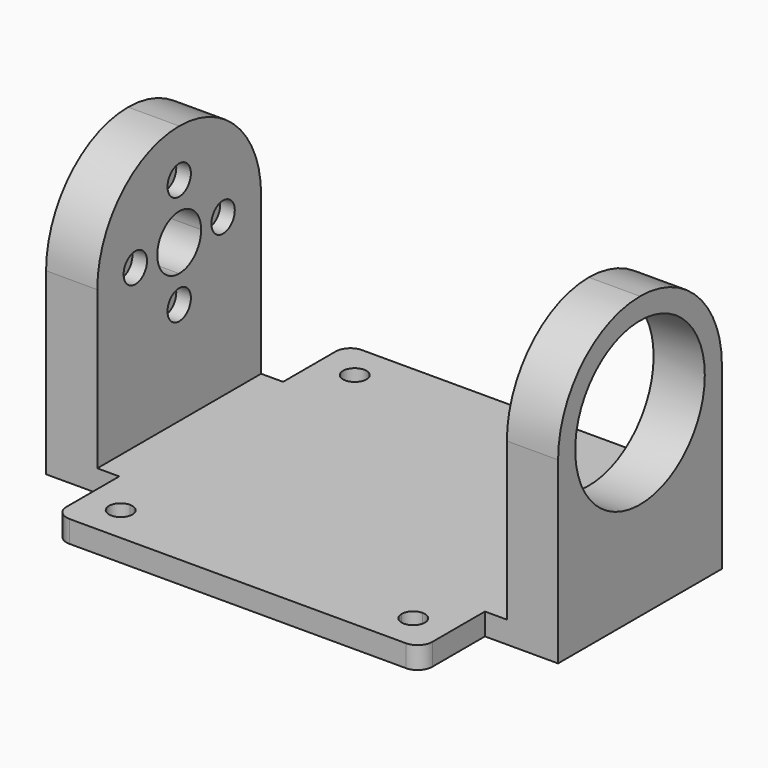
from build123d import *

# Parameters (mm, degrees)
F0_W      = 10
F0_H      = 14
F1_DEPTH  = 3
F2_W      = 7
F2_H      = 28
F3_DEPTH  = 35.5
F5_DEPTH  = 70.001
F6_R      = 11.075
F7_DEPTH  = 7
F9_DEPTH  = 25
F10_R     = 2
F11_DEPTH = 2


with BuildPart() as f1:
    # F0 (on Top) → F1 (new body)
    with BuildSketch(Plane.XY):
        with BuildLine():
            ThreePointArc((25, 23), (24.4142135624, 24.4142135624), (23, 25))
            Line((23, 25), (-23, 25))
            ThreePointArc((-23, 25), (-24.4142135624, 24.4142135624), (-25, 23))
            Line((-25, 23), (-25, 14))
            Line((-25, 14), (-25, 0))
            Line((-25, 0), (-25, -14))
            Line((-25, -14), (-25, -23))
            ThreePointArc((-25, -23), (-24.4142135624, -24.4142135624), (-23, -25))
            Line((-23, -25), (23, -25))
            ThreePointArc((23, -25), (24.4142135624, -24.4142135624), (25, -23))
            Line((25, -23), (25, -14))
            Line((25, -14), (25, 0))
            Line((25, 0), (25, 14))
            Line((25, 14), (25, 23))
        make_face()
        with BuildLine():
            ThreePointArc((-20, 18.4), (-21.1313708499, 21.1313708499), (-18.4, 20))
            Line((-18.4, 20), (18.4, 20))
            ThreePointArc((18.4, 20), (20, 21.6), (21.6, 20))
            ThreePointArc((21.6, 20), (21.1313708499, 18.8686291501), (20, 18.4))
            Line((20, 18.4), (20, -18.4))
            ThreePointArc((20, -18.4), (21.1313708499, -18.8686291501), (21.6, -20))
            ThreePointArc((21.6, -20), (20, -21.6), (18.4, -20))
            Line((18.4, -20), (-18.4, -20))
            ThreePointArc((-18.4, -20), (-21.1313708499, -21.1313708499), (-20, -18.4))
            Line((-20, -18.4), (-20, 18.4))
        make_face(mode=Mode.SUBTRACT)
        with Locations((30, 7)):
            Rectangle(F0_W, F0_H)
        with Locations((-30, 7)):
            Rectangle(F0_W, F0_H)
        with Locations((30, -7)):
            Rectangle(F0_W, F0_H)
        with Locations((-30, -7)):
            Rectangle(F0_W, F0_H)
        with BuildLine():
            Line((18.4, 20), (-18.4, 20))
            ThreePointArc((-18.4, 20), (-18.8686291501, 18.8686291501), (-20, 18.4))
            Line((-20, 18.4), (-20, -18.4))
            ThreePointArc((-20, -18.4), (-18.8686291501, -18.8686291501), (-18.4, -20))
            Line((-18.4, -20), (18.4, -20))
            ThreePointArc((18.4, -20), (18.8686291501, -18.8686291501), (20, -18.4))
            Line((20, -18.4), (20, 18.4))
            ThreePointArc((20, 18.4), (18.8686291501, 18.8686291501), (18.4, 20))
        make_face()
    extrude(amount=F1_DEPTH)

    # F2 (on face) → F3 (join)
    with BuildSketch(Plane.XY.offset(3)):
        with Locations((-31.5, 0)):
            Rectangle(F2_W, F2_H)
        with Locations((31.5, 0)):
            Rectangle(F2_W, F2_H)
    extrude(amount=F3_DEPTH)

    # F4 (on face) → F5 (cut, through all)
    with BuildSketch(Plane(origin=(-35, 0, 0), x_dir=(0, -1, 0), z_dir=(-1, 0, 0))):
        with BuildLine():
            Line((14, 38.5), (0, 38.5))
            ThreePointArc((0, 38.5), (9.8994949366, 34.3994949366), (14, 24.5))
            Line((14, 24.5), (14, 38.5))
        make_face()
        with BuildLine():
            ThreePointArc((-14, 24.5), (-9.8994949366, 34.3994949366), (0, 38.5))
            Line((0, 38.5), (-14, 38.5))
            Line((-14, 38.5), (-14, 24.5))
        make_face()
    extrude(amount=-F5_DEPTH, mode=Mode.SUBTRACT)

    # F6 (on face) → F7 (cut, through all)
    with BuildSketch(Plane.YZ.offset(35)):
        with Locations((0, 24.5)):
            Circle(F6_R)
    extrude(amount=-F7_DEPTH, mode=Mode.SUBTRACT)

    # F8 (on face) → F9 (cut)
    with BuildSketch(Plane(origin=(-35, 0, 0), x_dir=(0, -1, 0), z_dir=(-1, 0, 0))):
        with BuildLine():
            ThreePointArc((1, 32), (0.7071067812, 32.7071067812), (0, 33))
            Line((0, 33), (0, 32))
            ThreePointArc((0, 32), (0.5, 31.9833147735), (0.9977753031, 31.9333333333))
            ThreePointArc((0.9977753031, 31.9333333333), (0.999443671, 31.966648112), (1, 32))
        make_face()
        with BuildLine():
            Line((0, 32), (0, 33))
            ThreePointArc((0, 33), (-0.7302967433, 32.6831300511), (-0.9977753031, 31.9333333333))
            ThreePointArc((-0.9977753031, 31.9333333333), (-0.5, 31.9833147735), (0, 32))
        make_face()
        with BuildLine():
            Line((0, 31), (0, 32))
            ThreePointArc((0, 32), (-0.5, 31.9833147735), (-0.9977753031, 31.9333333333))
            ThreePointArc((-0.9977753031, 31.9333333333), (-0.6831300511, 31.2697032567), (0, 31))
        make_face()
        with BuildLine():
            ThreePointArc((0.9977753031, 31.9333333333), (0.5, 31.9833147735), (0, 32))
            Line((0, 32), (0, 31))
            ThreePointArc((0, 31), (0.6831300511, 31.2697032567), (0.9977753031, 31.9333333333))
        make_face()
        with BuildLine():
            ThreePointArc((-6.5, 24.5), (-6.7697032567, 25.1831300511), (-7.4333333333, 25.4977753031))
            ThreePointArc((-7.4333333333, 25.4977753031), (-7.4833147735, 25), (-7.5, 24.5))
            Line((-7.5, 24.5), (-6.5, 24.5))
        make_face()
        with BuildLine():
            ThreePointArc((-7.5, 24.5), (-7.4833147735, 25), (-7.4333333333, 25.4977753031))
            ThreePointArc((-7.4333333333, 25.4977753031), (-8.5, 24.5), (-7.4333333333, 23.5022246969))
            ThreePointArc((-7.4333333333, 23.5022246969), (-7.4833147735, 24), (-7.5, 24.5))
        make_face()
        with BuildLine():
            ThreePointArc((8.5, 24.5), (8.1831300511, 25.2302967433), (7.4333333333, 25.4977753031))
            ThreePointArc((7.4333333333, 25.4977753031), (7.4833147735, 25), (7.5, 24.5))
            ThreePointArc((7.5, 24.5), (7.4833147735, 24), (7.4333333333, 23.5022246969))
            ThreePointArc((7.4333333333, 23.5022246969), (8.1831300511, 23.7697032567), (8.5, 24.5))
        make_face()
        with BuildLine():
            ThreePointArc((7.5, 24.5), (7.4833147735, 25), (7.4333333333, 25.4977753031))
            ThreePointArc((7.4333333333, 25.4977753031), (6.7697032567, 25.1831300511), (6.5, 24.5))
            Line((6.5, 24.5), (7.5, 24.5))
        make_face()
        with BuildLine():
            ThreePointArc((3.75, 24.5), (2.6516504294, 27.1516504294), (0, 28.25))
            Line((0, 28.25), (0, 24.5))
            Line((0, 24.5), (3.75, 24.5))
        make_face()
        with BuildLine():
            Line((0, 24.5), (0, 28.25))
            ThreePointArc((0, 28.25), (-2.6516504294, 27.1516504294), (-3.75, 24.5))
            Line((-3.75, 24.5), (0, 24.5))
        make_face()
        with BuildLine():
            Line((-6.5, 24.5), (-7.5, 24.5))
            ThreePointArc((-7.5, 24.5), (-7.4833147735, 24), (-7.4333333333, 23.5022246969))
            ThreePointArc((-7.4333333333, 23.5022246969), (-6.7697032567, 23.8168699489), (-6.5, 24.5))
        make_face()
        with BuildLine():
            ThreePointArc((7.4333333333, 23.5022246969), (7.4833147735, 24), (7.5, 24.5))
            Line((7.5, 24.5), (6.5, 24.5))
            ThreePointArc((6.5, 24.5), (6.7697032567, 23.8168699489), (7.4333333333, 23.5022246969))
        make_face()
        with BuildLine():
            Line((3.75, 24.5), (0, 24.5))
            Line((0, 24.5), (0, 20.75))
            ThreePointArc((0, 20.75), (2.6516504294, 21.8483495706), (3.75, 24.5))
        make_face()
        with BuildLine():
            Line((0, 20.75), (0, 24.5))
            Line((0, 24.5), (-3.75, 24.5))
            ThreePointArc((-3.75, 24.5), (-2.6516504294, 21.8483495706), (0, 20.75))
        make_face()
        with BuildLine():
            ThreePointArc((0, 18), (-0.6831300511, 17.7302967433), (-0.9977753031, 17.0666666667))
            ThreePointArc((-0.9977753031, 17.0666666667), (-0.5, 17.0166852265), (0, 17))
            Line((0, 17), (0, 18))
        make_face()
        with BuildLine():
            ThreePointArc((0, 17), (-0.5, 17.0166852265), (-0.9977753031, 17.0666666667))
            ThreePointArc((-0.9977753031, 17.0666666667), (-0.033351888, 16.000556329), (1, 17))
            ThreePointArc((1, 17), (0.999443671, 17.033351888), (0.9977753031, 17.0666666667))
            ThreePointArc((0.9977753031, 17.0666666667), (0.5, 17.0166852265), (0, 17))
        make_face()
        with BuildLine():
            Line((0, 18), (0, 17))
            ThreePointArc((0, 17), (0.5, 17.0166852265), (0.9977753031, 17.0666666667))
            ThreePointArc((0.9977753031, 17.0666666667), (0.6831300511, 17.7302967433), (0, 18))
        make_face()
    extrude(amount=-F9_DEPTH, mode=Mode.SUBTRACT)

    # F10 (on face) → F11 (cut)
    with BuildSketch(Plane.YZ.offset(-28)):
        with Locations((-7.5, 24.5)):
            Circle(F10_R)
        with Locations((0, 17)):
            Circle(F10_R)
        with Locations((0, 32)):
            Circle(F10_R)
        with Locations((7.5, 24.5)):
            Circle(F10_R)
    extrude(amount=-F11_DEPTH, mode=Mode.SUBTRACT)


solid = f1.part
